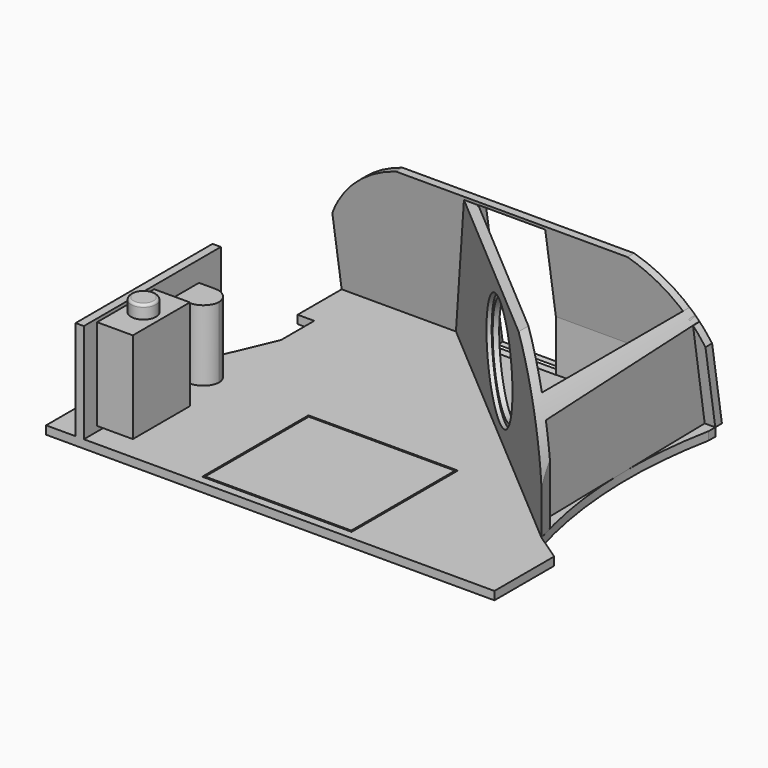
from build123d import *

# Parameters (mm, degrees)
F1_DEPTH     = 25.4
F2_W         = 457.2
F2_H         = 406.4
F3_DEPTH     = 25.4
F4_W         = 447.04
F4_H         = 396.24
F5_DEPTH     = 25.4
F7_DEPTH     = 1143
F9_DEPTH     = 406.4
F11_DEPTH    = 1143
F12_R        = 165.1
F13_DEPTH    = 12.7
F14_R        = 152.4
F15_DEPTH    = 25.4
F16_W        = 203.2
F16_H        = 414.02
F17_DEPTH    = 50.8
F19_DEPTH    = 990.6
F21_DEPTH    = 304.8
F22_W        = 218.44
F22_H        = 279.4
F23_DEPTH    = 109.22
F24_R        = 38.1
F25_DEPTH    = 40.64
F26_R        = 7.62
F27_W        = 95.25
F27_H        = 216.662
F28_DEPTH    = 99.822
F29_T1_DEPTH = 343.662


# Not quite as in the source:
# - a fillet or chamfer that OpenCascade refuses, or shapes differently, is made with other operations: its cross-section is extruded or revolved along the edge and cut away or added


with BuildPart() as f1:
    # F0 (on Top) → F1 (new body)
    with BuildSketch(Plane.XY):
        with BuildLine():
            Line((568.96, 381), (-574.04, 381))
            Line((-574.04, 381), (-574.04, 212.5894725323))
            Line((-574.04, 212.5894725323), (-523.24, 212.5894725323))
            Line((-523.24, 212.5894725323), (-523.24, 85.5894725323))
            Line((-523.24, 85.5894725323), (-595.9868865448, -85.3224374884))
            Line((-595.9868865448, -85.3224374884), (-595.8204893284, -288.5223693584))
            Line((-595.8204893284, -288.5223693584), (-685.8, -304.8))
            Line((-685.8, -304.8), (-685.8, -609.6))
            Line((-685.8, -609.6), (685.8, -609.6))
            Line((685.8, -609.6), (685.8, -381))
            Line((685.8, -381), (601.5101489935, -324.2745117491))
            ThreePointArc((601.5101489935, -324.2745117491), (543.9222330335, 13.6848215504), (568.96, 355.6))
            Line((568.96, 355.6), (568.96, 381))
        make_face()
    extrude(amount=F1_DEPTH)

    # F2 (on face) → F3 (cut)
    with BuildSketch(Plane.XY.offset(25.4)):
        with Locations((0, -381)):
            Rectangle(F2_W, F2_H)
    extrude(amount=-F3_DEPTH, mode=Mode.SUBTRACT)


with BuildPart() as f5:
    # F4 (on face) → F5 (new body)
    with BuildSketch(Plane.XY.offset(25.4)):
        with Locations((0, -381)):
            Rectangle(F4_W, F4_H)
    extrude(amount=-F5_DEPTH)


with BuildPart() as f7:
    # F6 (on face) → F7 (new body)
    with BuildSketch(Plane(origin=(-574.04, 0, 0), x_dir=(0, -1, 0), z_dir=(-1, 0, 0))):
        Polygon((-406.4, 25.4), (-381, 25.4), (-313.450360893, 441.593868115), (-338.850360893, 441.593868115), align=None)
    extrude(amount=-F7_DEPTH)


with BuildPart() as f9:
    # F8 (on face) → F9 (new body)
    with BuildSketch(Plane.XY.offset(25.4)):
        Polygon((601.5101489935, -324.2745117491), (587.793108051, -275.0426883363), (549.0162910079, -241.9296818818), (536.6005640478, 381), (511.2005640478, 381), (-180.4623305798, 381), (-224.3979649328, 381), align=None)
        Polygon((511.2005640478, -209.6373869903), (-150.7177903415, 355.6), (511.2005640478, 355.6), align=None, mode=Mode.SUBTRACT)
    extrude(amount=F9_DEPTH)

    # F10 (on face) → F11 (cut)
    with BuildSketch(Plane(origin=(-574.04, 0, 0), x_dir=(0, -1, 0), z_dir=(-1, 0, 0))):
        Polygon((-401.2590646744, 460.1649348316), (-406.4, 25.4), (-335.8362154414, 460.1649348316), align=None)
    extrude(amount=-F11_DEPTH, mode=Mode.SUBTRACT)

    # F12 (on face) → F13 (cut)
    with BuildSketch(Plane(origin=(93.5207792511, 109.5170307696, 0), x_dir=(0.7604594625, -0.6493854063, 0), z_dir=(-0.6493854063, -0.7604594625, 0))):
        with Locations((134.6032201509, 228.6)):
            Circle(F12_R)
    extrude(amount=-F13_DEPTH, mode=Mode.SUBTRACT)

    # F14 (on face) → F15 (cut)
    with BuildSketch(Plane(origin=(101.767973911, 119.1748659433, 0), x_dir=(0.7604594625, -0.6493854063, 0), z_dir=(-0.6493854063, -0.7604594625, 0))):
        with Locations((134.6032201509, 228.6)):
            Circle(F14_R)
    extrude(amount=-F15_DEPTH, mode=Mode.SUBTRACT)


with BuildPart() as f17_tool:
    # F16 (on face) → F17 (new body)
    with BuildSketch(Plane(origin=(0, 399.9859297679, 64.9190371931), x_dir=(-1, 0, 0), z_dir=(0, 0.9870834554, 0.1602069042))):
        with Locations((0, 169.5138338797)):
            Rectangle(F16_W, F16_H)
    extrude(amount=-F17_DEPTH)


with BuildPart() as f1_1:
    add(f1.part)

    # F17: cut by f17_tool
    add(f17_tool.part, mode=Mode.SUBTRACT)

    # F20 (on face) → F21 (join)
    with BuildSketch(Plane.XY.offset(25.4)):
        Polygon((-570.2823618796, -609.6), (-570.5868865448, -85.3224374884), (-595.9868865448, -85.3224374884), (-595.5575639255, -609.6), align=None)
    extrude(amount=F21_DEPTH)

    # F22 (on face) → F23 (join)
    with BuildSketch(Plane(origin=(-570.6362532415, -0.3314519377, 0), x_dir=(-0.0005808462, 0.9999998313, 0), z_dir=(0.9999998313, 0.0005808462, 0))):
        with Locations((-449.2486508406, 180.34)):
            Rectangle(F22_W, F22_H)
    extrude(amount=F23_DEPTH)

    # F24 (on face) → F25 (join)
    with BuildSketch(Plane.XY.offset(320.04)):
        with Locations((-515.8287581144, -449.5165869753)):
            Circle(F24_R)
    extrude(amount=F25_DEPTH)

    # F26
    f26_edges = [f1_1.edges().sort_by_distance(p)[0] for p in [
        (-553.928758, -449.516587, 360.68),
    ]]
    fillet(f26_edges, radius=F26_R)

    # F27 (on face) → F28 (join)
    with BuildSketch(Plane(origin=(-570.6362532415, -0.3314519377, 0), x_dir=(-0.0005808462, 0.9999998313, 0), z_dir=(0.9999998313, 0.0005808462, 0))):
        with Locations((-216.2036508406, 159.131)):
            Rectangle(F27_W, F27_H)
    extrude(amount=F28_DEPTH)

    # F29: fillet of radius 50.8 on 2 edges, made by hand

    # F29_s2 → F29_t1 (cut)
    with BuildSketch(Plane.XY.offset(50.8)):
        with BuildLine():
            ThreePointArc((-521.5163432475, -168.8816000996), (-485.5866824268, -183.7397085159), (-470.6868448316, -219.6520845447))
            Line((-470.6868448316, -219.6520845447), (-470.716351817, -168.8520931142))
            Line((-470.716351817, -168.8520931142), (-521.5163432475, -168.8816000996))
        make_face()
        with BuildLine():
            ThreePointArc((-521.4610176499, -264.1315840318), (-485.5486416211, -249.2317464365), (-470.6905332048, -213.3020856159))
            Line((-470.6905332048, -213.3020856159), (-470.6610262194, -264.1020770464))
            Line((-470.6610262194, -264.1020770464), (-521.4610176499, -264.1315840318))
        make_face()
    extrude(amount=F29_T1_DEPTH, mode=Mode.SUBTRACT)


with BuildPart() as f7_1:
    add(f7.part)

    # F17: cut by f17_tool
    add(f17_tool.part, mode=Mode.SUBTRACT)


with BuildPart() as f9_1:
    add(f9.part)

    # F17: cut by f17_tool
    add(f17_tool.part, mode=Mode.SUBTRACT)


with BuildPart() as f19_tool:
    # F18 (on face) → F19 (new body)
    with BuildSketch(Plane.XZ.offset(609.6)):
        with BuildLine():
            Line((605.9201579013, 445.1687633991), (566.9001340866, 445.1687633991))
            Line((566.9001340866, 445.1687633991), (342.9, 445.1687633991))
            ThreePointArc((342.9, 445.1687633991), (522.2177920978, 327.696172597), (605.9201579013, 130.3421908498))
            Line((605.9201579013, 130.3421908498), (605.9201579013, 235.2843816996))
            Line((605.9201579013, 235.2843816996), (605.9201579013, 445.1687633991))
        make_face()
        with BuildLine():
            Line((-342.9, 445.1687633991), (-566.9001340866, 445.1687633991))
            Line((-566.9001340866, 445.1687633991), (-605.9201579013, 445.1687633991))
            Line((-605.9201579013, 445.1687633991), (-605.9201579013, 235.2843816996))
            Line((-605.9201579013, 235.2843816996), (-605.9201579013, 130.3421908498))
            ThreePointArc((-605.9201579013, 130.3421908498), (-522.2177920978, 327.696172597), (-342.9, 445.1687633991))
        make_face()
    extrude(amount=-F19_DEPTH)


with BuildPart() as f7_2:
    add(f7_1.part)

    # F19: cut by f19_tool
    add(f19_tool.part, mode=Mode.SUBTRACT)


with BuildPart() as f9_2:
    add(f9_1.part)

    # F19: cut by f19_tool
    add(f19_tool.part, mode=Mode.SUBTRACT)


solid = Compound([f5.part, f1_1.part, f7_2.part, f9_2.part])
